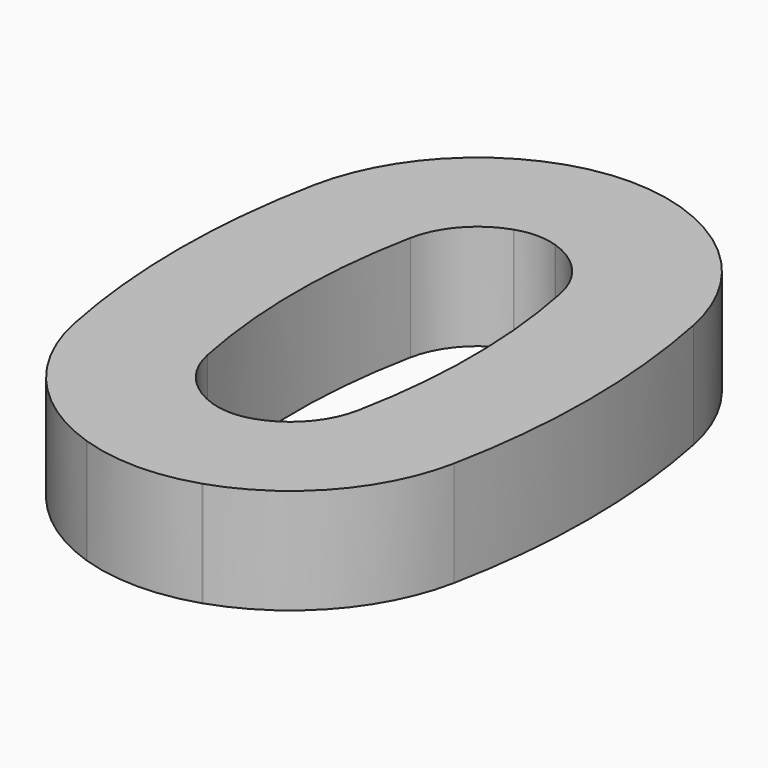
from build123d import *

# Parameters (mm, degrees)
F1_DEPTH    = 4.5
F2_R        = 17
F3_T1_DEPTH = 33.9045095963
F5_DEPTH    = 9


# Not quite as in the source:
# - a fillet or chamfer that OpenCascade refuses, or shapes differently, is made with other operations: its cross-section is extruded or revolved along the edge and cut away or added


with BuildPart() as f1:
    # F0 (on Top) → F1 (new body, symmetric)
    with BuildSketch(Plane.XY):
        with BuildLine():
            ThreePointArc((15.375, -16.5), (17.5041005313, 0), (15.375, 16.5))
            ThreePointArc((15.375, 16.5), (9.0566864996, 23.6051242432), (0, 26.5))
            ThreePointArc((0, 26.5), (-9.0566864996, 23.6051242432), (-15.375, 16.5))
            ThreePointArc((-15.375, 16.5), (-17.5041005313, 0), (-15.375, -16.5))
            ThreePointArc((-15.375, -16.5), (-9.0566864996, -23.6051242432), (0, -26.5))
            ThreePointArc((0, -26.5), (9.0566864996, -23.6051242432), (15.375, -16.5))
        make_face()
    extrude(amount=F1_DEPTH, both=True)

    # F2
    f2_edges = [f1.edges().sort_by_distance(p)[0] for p in [
        (-15.375, 16.5, 0),
        (-15.375, -16.5, 0),
        (15.375, -16.5, 0),
        (15.375, 16.5, 0),
    ]]
    fillet(f2_edges, radius=F2_R)

    # F3: fillet of radius 15.59 on 2 edges, made by hand

    # F3_s2 → F3_t1 (cut)
    with BuildSketch(Plane.XY.offset(-16.9522547982)):
        with BuildLine():
            ThreePointArc((4.8996291219, 25.603887062), (0, 26.3938284652), (-4.8996291219, 25.603887062))
            ThreePointArc((-4.8996291219, 25.603887062), (-2.4809605234, 26.222238656), (0, 26.5))
            ThreePointArc((0, 26.5), (2.4809605234, 26.222238656), (4.8996291219, 25.603887062))
        make_face()
        with BuildLine():
            ThreePointArc((4.8996291219, -25.603887062), (0, -26.3938284652), (-4.8996291219, -25.603887062))
            ThreePointArc((-4.8996291219, -25.603887062), (-2.4809605234, -26.222238656), (0, -26.5))
            ThreePointArc((0, -26.5), (2.4809605234, -26.222238656), (4.8996291219, -25.603887062))
        make_face()
    extrude(amount=F3_T1_DEPTH, mode=Mode.SUBTRACT)

    # F4 (on face) → F5 (cut, through all)
    with BuildSketch(Plane.XY.offset(4.5)):
        with BuildLine():
            ThreePointArc((-6.424547387, 10.8436806891), (-7.5041005313, 0), (-6.424547387, -10.8436806891))
            ThreePointArc((-6.424547387, -10.8436806891), (-4.8148810997, -14.0903093829), (-1.797468323, -16.0970090531))
            ThreePointArc((-1.797468323, -16.0970090531), (-1.7771565537, -16.1038240182), (-1.7568266062, -16.1105845625))
            ThreePointArc((-1.7568266062, -16.1105845625), (0, -16.3938284652), (1.7568266062, -16.1105845625))
            ThreePointArc((1.7568266062, -16.1105845625), (1.7771565537, -16.1038240182), (1.797468323, -16.0970090531))
            ThreePointArc((1.797468323, -16.0970090531), (4.8148810997, -14.0903093829), (6.424547387, -10.8436806891))
            ThreePointArc((6.424547387, -10.8436806891), (7.5041005313, 0), (6.424547387, 10.8436806891))
            ThreePointArc((6.424547387, 10.8436806891), (4.8148810997, 14.0903093829), (1.797468323, 16.0970090531))
            ThreePointArc((1.797468323, 16.0970090531), (1.7771565537, 16.1038240182), (1.7568266062, 16.1105845625))
            ThreePointArc((1.7568266062, 16.1105845625), (0, 16.3938284652), (-1.7568266062, 16.1105845625))
            ThreePointArc((-1.7568266062, 16.1105845625), (-1.7771565537, 16.1038240182), (-1.797468323, 16.0970090531))
            ThreePointArc((-1.797468323, 16.0970090531), (-4.8148810997, 14.0903093829), (-6.424547387, 10.8436806891))
        make_face()
    extrude(amount=-F5_DEPTH, mode=Mode.SUBTRACT)


solid = f1.part
